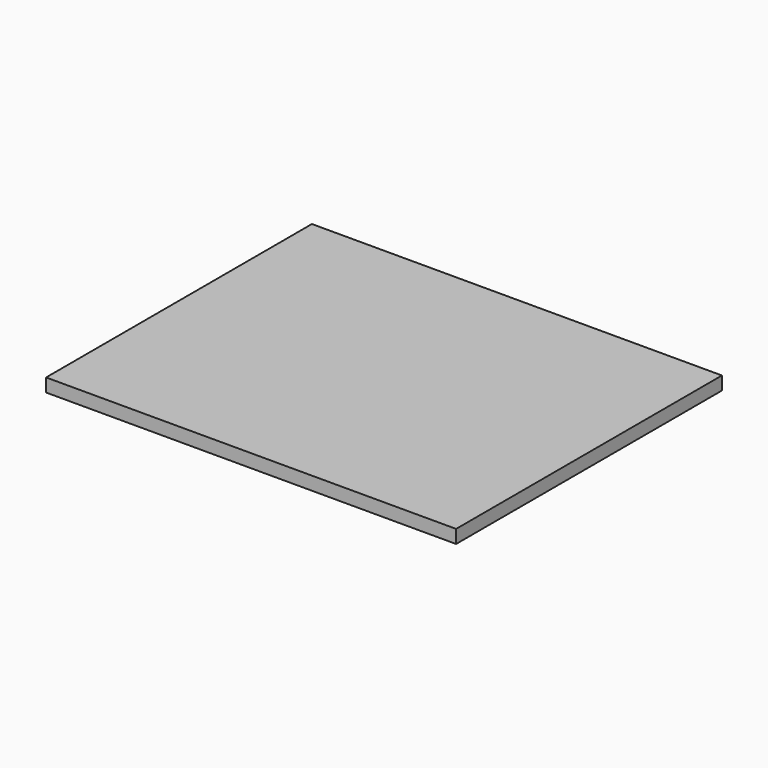
from build123d import *

# Parameters (mm, degrees)
F0_W     = 78.3598385751
F0_H     = 72.739217896
F0_R     = 13.705932092
F0_R_2   = 10.2154908805
F1_DEPTH = 63.5
F2_T     = 2.54


# Not quite as in the source:
# - a shell that OpenCascade refuses in one call is made with other operations: the cavity is built on its own and cut out


with BuildPart() as f1:
    # F0 (on Front) → F1 (new body)
    with BuildSketch(Plane.XZ):
        with Locations((3.2207649201, 1.5117155854)):
            Rectangle(F0_W, F0_H)
        with Locations((18.9568325877, -4.6814545058)):
            Circle(F0_R, mode=Mode.SUBTRACT)
        with Locations((-12.9959195619, 25.2717551775)):
            Circle(F0_R_2, mode=Mode.SUBTRACT)
        with Locations((18.9568325877, -4.6814545058)):
            Circle(F0_R)
    extrude(amount=F1_DEPTH)

    # F2: shell of thickness 2.54, made by hand


with BuildPart() as f2_core1:
    # F2_t2: copy of F1
    add(f1.part)

    # the walls: a layer under each face that stays
    f2_faces = [f2_core1.faces().sort_by_distance(p)[0] for p in [
        (3.2207649201, -31.75, -34.8578933626),
    ]]
    thicken(f2_faces, amount=-F2_T, mode=Mode.SUBTRACT)


with BuildPart() as f1_1:
    add(f1.part)

    # what is left inside the walls is the cavity
    f2_cavity = [f2_core1.part.solids().sort_by_distance(p)[0] for p in [
        (3.220765, -0.0254, -8.918154),
    ]]
    add(f2_cavity, mode=Mode.SUBTRACT)


solid = f1_1.part
